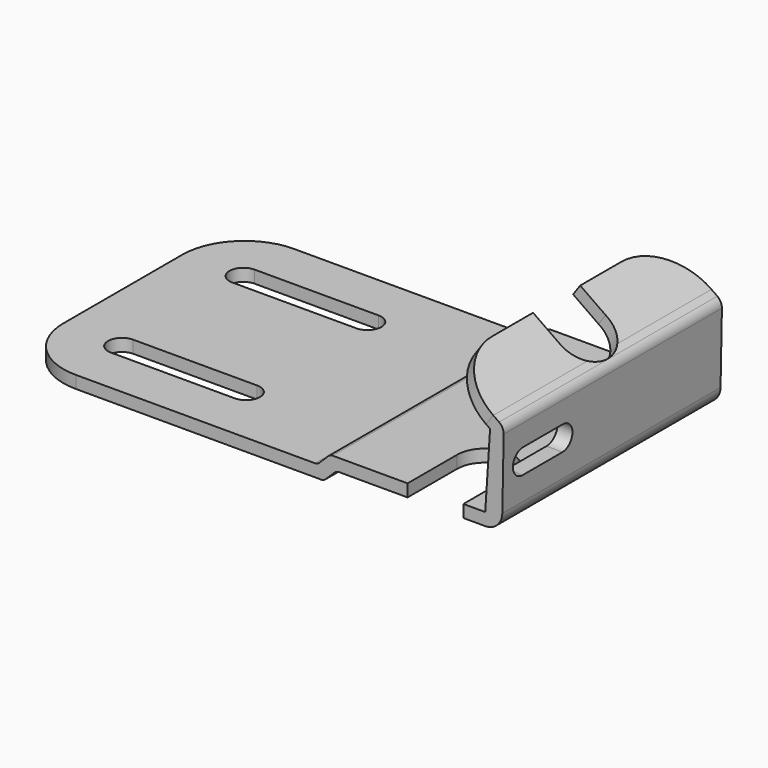
from build123d import *

# Parameters (mm, degrees)
F1_DEPTH  = 22
F3_DEPTH  = 2
F5_DEPTH  = 25
F7_DEPTH  = 25
F9_DEPTH  = 2
F11_DEPTH = 2.4954547296
F13_DEPTH = 2
F14_DEPTH = 25


# Not quite as in the source:
# - a feature names something its author has since deleted; it is built from what else it names


with BuildPart() as f1:
    # F0 (on Front) → F1 (new body, symmetric)
    with BuildSketch(Plane.XZ):
        with BuildLine():
            Line((-40, 0), (-0.4058661959, 0))
            ThreePointArc((-0.4058661959, 0), (-0.0297944203, 0.073409465), (0.2910628996, 0.2828599608))
            Line((0.2910628996, 0.2828599608), (1.7669371004, 1.7171400392))
            ThreePointArc((1.7669371004, 1.7171400392), (2.0877944203, 1.926590535), (2.4638661959, 2))
            Line((2.4638661959, 2), (26.037, 2))
            ThreePointArc((26.037, 2), (27.9687843496, 2.7891547709), (28.7954749436, 4.705176349))
            Line((28.7954749436, 4.705176349), (29.016465998, 16.0310205539))
            ThreePointArc((29.016465998, 16.0310205539), (28.8276722638, 16.8546583092), (28.2736767263, 17.4927109486))
            Line((28.2736767263, 17.4927109486), (27.3333525812, 18.1512658075))
            Line((27.3333525812, 18.1512658075), (26.1860444646, 16.5130704329))
            Line((26.1860444646, 16.5130704329), (26.8254471929, 16.0652655182))
            Line((26.8254471929, 16.0652655182), (26.037, 4))
            Line((26.037, 4), (1.4428661959, 4))
            ThreePointArc((1.4428661959, 4), (1.0667944203, 3.926590535), (0.7459371004, 3.7171400392))
            Line((0.7459371004, 3.7171400392), (-0.7299371004, 2.2828599608))
            ThreePointArc((-0.7299371004, 2.2828599608), (-1.0507944203, 2.073409465), (-1.4268661959, 2))
            Line((-1.4268661959, 2), (-40, 2))
            Line((-40, 2), (-40, 0))
        make_face()
    extrude(amount=F1_DEPTH, both=True)

    # F2 (on face) → F3 (join)
    with BuildSketch(Plane.XY.offset(2)):
        with BuildLine():
            Line((-50, 12), (-50, -12))
            ThreePointArc((-50, -12), (-47.0710678119, -19.0710678119), (-40, -22))
            Line((-40, -22), (-40, 22))
            ThreePointArc((-40, 22), (-47.0710678119, 19.0710678119), (-50, 12))
        make_face()
    extrude(amount=-F3_DEPTH)

    # F4 (on face) → F5 (cut)
    with BuildSketch(Plane.XY.offset(2)):
        with BuildLine():
            ThreePointArc((-40.35, 14.489), (-42.6, 12.239), (-40.35, 9.989))
            Line((-40.35, 9.989), (-20.35, 9.989))
            ThreePointArc((-20.35, 9.989), (-18.1, 12.239), (-20.35, 14.489))
            Line((-20.35, 14.489), (-40.35, 14.489))
        make_face()
    extrude(amount=-F5_DEPTH, mode=Mode.SUBTRACT)

    # F6 (on face) → F7 (cut)
    with BuildSketch(Plane(origin=(28.6927430868, 0, -0.5598557981), x_dir=(0, 1, 0), z_dir=(0.9998096932, 0, -0.0195083911))):
        with BuildLine():
            Line((-9.9999997095, 13.096034309), (-17.9999997095, 13.096034309))
            ThreePointArc((-17.9999997095, 13.096034309), (-20, 11.0960344543), (-18, 9.096034309))
            Line((-18, 9.096034309), (-9.9999997095, 9.096034309))
            ThreePointArc((-9.9999997095, 9.096034309), (-7.9999997095, 11.096034309), (-9.9999997095, 13.096034309))
        make_face()
    extrude(amount=-F7_DEPTH, mode=Mode.SUBTRACT)

    # F8 (on face) → F9 (join)
    with BuildSketch(Plane(origin=(17.5237251574, 0, 25.0214263138), x_dir=(0.8190976873, 0, -0.5736540583), z_dir=(0.5736540583, 0, 0.8190976873))):
        with BuildLine():
            Line((2.9761385921, 13), (2.9761385921, -13))
            ThreePointArc((2.9761385921, -13), (5.6121775614, -19.3639610307), (11.9761385921, -22))
            Line((11.9761385921, -22), (11.9761385921, 22))
            ThreePointArc((11.9761385921, 22), (5.6121775614, 19.3639610307), (2.9761385921, 13))
        make_face()
    extrude(amount=-F9_DEPTH)

    # F10 (on face) → F11 (cut, through all)
    with BuildSketch(Plane(origin=(17.5237251574, 0, 25.0214263138), x_dir=(0.8190976873, 0, -0.5736540583), z_dir=(0.5736540583, 0, 0.8190976873))):
        with BuildLine():
            Line((2.9761385921, 4.75), (2.9761385921, -4.75))
            Line((2.9761385921, -4.75), (7.9761385921, -4.75))
            ThreePointArc((7.9761385921, -4.75), (13.0569949576, 0), (7.9761385921, 4.75))
            Line((7.9761385921, 4.75), (2.9761385921, 4.75))
        make_face()
    extrude(amount=-F11_DEPTH, mode=Mode.SUBTRACT)

    # F12 (on face) → F13 (cut, through all)
    with BuildSketch(Plane(origin=(0, 0, 2), x_dir=(1, 0, 0), z_dir=(0, 0, -1))):
        with BuildLine():
            Line((22.517, 12), (22.517, 22))
            Line((22.517, 22), (13.517, 22))
            Line((13.517, 22), (13.517, 12))
            ThreePointArc((13.517, 12), (18.017, 7.5), (22.517, 12))
        make_face()
    extrude(amount=-F13_DEPTH, mode=Mode.SUBTRACT)

    # F4 (on face) → F14 (cut)
    with BuildSketch(Plane.XY.offset(2)):
        with BuildLine():
            Line((-20.35, -9.989), (-40.35, -9.989))
            ThreePointArc((-40.35, -9.989), (-42.6, -12.239), (-40.35, -14.489))
            Line((-40.35, -14.489), (-20.35, -14.489))
            ThreePointArc((-20.35, -14.489), (-18.1, -12.239), (-20.35, -9.989))
        make_face()
    extrude(amount=-F14_DEPTH, mode=Mode.SUBTRACT)


solid = f1.part
